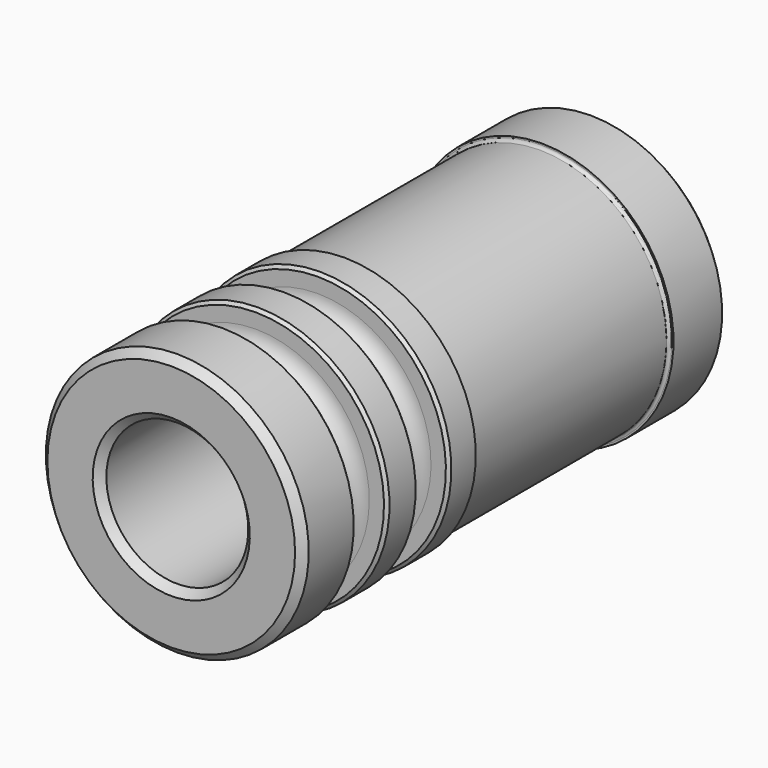
from build123d import *

# Parameters (mm, degrees)
F3_SIZE = 0.635
F4_SIZE = 0.254


# Not quite as in the source:
# - a fillet or chamfer that OpenCascade refuses, or shapes differently, is made with other operations: its cross-section is extruded or revolved along the edge and cut away or added
# - ends of sketch curves that miss each other by under 0.0002 mm in the source are joined


with BuildPart() as f1:
    # F0 (on Right) → F1 (revolve)
    with BuildSketch(Plane.YZ):
        with BuildLine():
            Line((22.2140969225, 8.255), (22.2140969225, 10.9855))
            Line((22.2140969225, 10.9855), (16.4990969225, 10.9855))
            Line((16.4990969225, 10.9855), (16.4990969225, 10.8495159149))
            ThreePointArc((16.4990969225, 10.8495159149), (16.4273334225, 10.6762635), (16.2540810076, 10.6045))
            Line((16.2540810076, 10.6045), (-3.9060871626, 10.6045))
            ThreePointArc((-3.9060871626, 10.6045), (-4.0793395775, 10.6762635), (-4.1511030775, 10.8495159149))
            Line((-4.1511030775, 10.8495159149), (-4.1511030775, 10.9855))
            Line((-4.1511030775, 10.9855), (-6.9578040841, 10.9855))
            Line((-6.9578040841, 10.9855), (-6.9578040841, 9.4869))
            ThreePointArc((-6.9578040841, 9.4869), (-7.4302115567, 8.3464074726), (-8.5707040841, 7.874))
            ThreePointArc((-8.5707040841, 7.874), (-9.7111966115, 8.3464074726), (-10.1836040841, 9.4869))
            Line((-10.1836040841, 9.4869), (-10.1836040841, 10.9855))
            Line((-10.1836040841, 10.9855), (-13.4221030775, 10.9855))
            Line((-13.4221030775, 10.9855), (-13.4221030775, 9.49706))
            ThreePointArc((-13.4221030775, 9.49706), (-13.8826805689, 8.3507887918), (-15.0223040841, 7.874))
            Line((-15.0223040841, 7.874), (-15.0241, 7.874))
            ThreePointArc((-15.0241, 7.874), (-16.1717722238, 8.3501225728), (-16.6479030775, 9.4977909507))
            Line((-16.6479030775, 9.4977909507), (-16.6479030775, 10.9855))
            Line((-16.6479030775, 10.9855), (-22.2359030775, 10.9855))
            Line((-22.2359030775, 10.9855), (-22.2359030775, 5.9309))
            Line((-22.2359030775, 5.9309), (-6.9959030775, 5.9309))
            Line((-6.9959030775, 5.9309), (-6.9959030775, 7.2009))
            Line((-6.9959030775, 7.2009), (-3.1859030775, 7.2009))
            Line((-3.1859030775, 7.2009), (-3.1859030775, 5.9309))
            Line((-3.1859030775, 5.9309), (-3.1859030775, 4.1275))
            Line((-3.1859030775, 4.1275), (0.6240969225, 4.1275))
            Line((0.6240969225, 4.1275), (22.2140969225, 8.255))
        make_face()
    revolve(axis=Axis((0, -0.0109030775, 0), (0, 1, 0)))

    # F2: chamfer of 0.635 on 2 edges, made by hand

    # F2_s1 → F2_t2 (revolve, cut)
    with BuildSketch(Plane.YZ):
        Polygon((21.6983345602, 8.1563983719), (22.2140969225, 8.780102938), (22.2140969225, 8.255), align=None)
    revolve(axis=Axis((0, 22.2140969225, 0), (0, 1, 0)), mode=Mode.SUBTRACT)

    # F2_s3 → F2_t4 (revolve, cut)
    with BuildSketch(Plane.YZ):
        Polygon((22.2140969225, 10.3505), (21.5790969225, 10.9855), (22.2140969225, 10.9855), align=None)
    revolve(axis=Axis((0, 22.2140969225, 0), (0, 1, 0)), mode=Mode.SUBTRACT)

    # F3
    f3_edges = [f1.edges().sort_by_distance(p)[0] for p in [
        (0, -22.235903, -10.9855),
        (0, -22.235903, -5.9309),
    ]]
    chamfer(f3_edges, length=F3_SIZE)

    # F4
    f4_edges = [f1.edges().sort_by_distance(p)[0] for p in [
        (0, -6.957804, -10.9855),
        (0, -13.422103, -10.9855),
        (0, -16.647903, -10.9855),
        (0, -10.183604, -10.9855),
    ]]
    chamfer(f4_edges, length=F4_SIZE)


solid = f1.part
